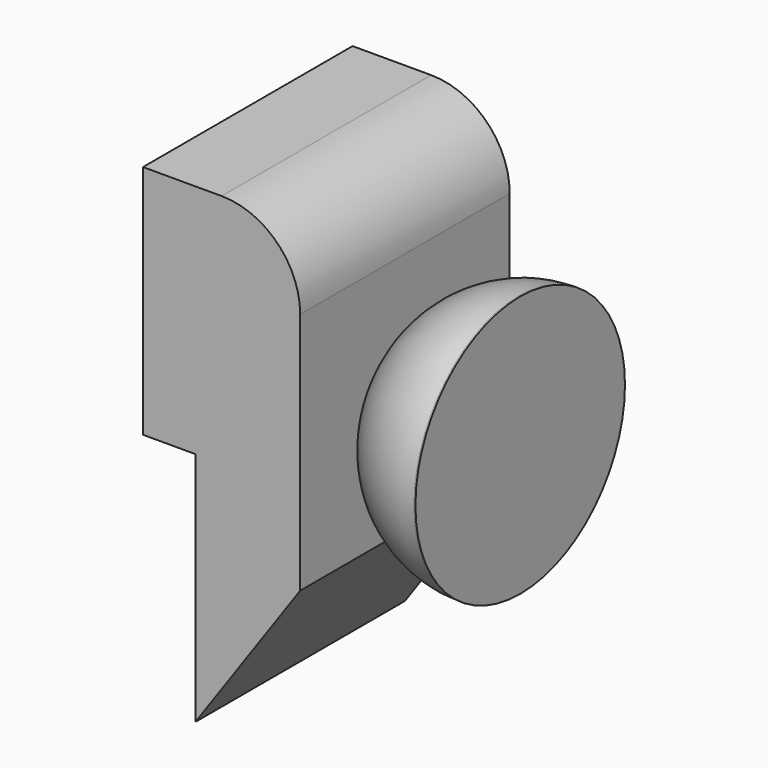
from build123d import *

# Parameters (mm, degrees)
F0_W      = 127
F0_H      = 228.6
F1_DEPTH  = 50.8
F2_R      = 38.1
F3_SIZE2  = 72.549909
F3_SIZE   = 50.79999
F4_W      = 127
F4_H      = 12.7
F5_DEPTH  = 25.4
F6_W      = 127
F6_H      = 101.6
F7_DEPTH  = 25.4
F8_R      = 25.4
F9_DEPTH  = 1.27
F10_R     = 63.5
F11_DEPTH = 54.61


# Not quite as in the source:
# - a fillet or chamfer that OpenCascade refuses, or shapes differently, is made with other operations: its cross-section is extruded or revolved along the edge and cut away or added
# - a fillet or chamfer is up to 0.001 mm smaller than in the source, because OpenCascade refuses the exact size


with BuildPart() as f1:
    # F0 (on Right) → F1 (new body)
    with BuildSketch(Plane.YZ):
        Rectangle(F0_W, F0_H)
    extrude(amount=F1_DEPTH)

    # F2
    f2_edges = [f1.edges().sort_by_distance(p)[0] for p in [
        (50.8, 0, 114.3),
    ]]
    fillet(f2_edges, radius=F2_R)

    # F3 (size 50.8 and 72.5499187425 in the source; OpenCascade refuses exactly that, so slightly less here)
    f3_edges = [f1.edges().sort_by_distance(p)[0] for p in [
        (50.8, 0, -114.3),
    ]]
    f3_side = f1.faces().sort_by_distance((25.4, 0, -114.3))[0]
    chamfer(f3_edges, length=F3_SIZE, length2=F3_SIZE2, reference=f3_side)

    # F4 (on face) → F5 (join)
    with BuildSketch(Plane(origin=(0, 0, 0), x_dir=(0, -1, 0), z_dir=(-1, 0, 0))):
        with Locations((0, 107.95)):
            Rectangle(F4_W, F4_H)
    extrude(amount=F5_DEPTH)

    # F6 (on face) → F7 (join)
    with BuildSketch(Plane(origin=(0, 0, 0), x_dir=(0, -1, 0), z_dir=(-1, 0, 0))):
        with Locations((0, 50.8)):
            Rectangle(F6_W, F6_H)
    extrude(amount=F7_DEPTH)

    # F8 (on face) → F9 (join)
    with BuildSketch(Plane.YZ.offset(50.8)):
        with Locations((0, 12.7)):
            Circle(F8_R)
    extrude(amount=F9_DEPTH)

    # F10 (on face) → F11 (join)
    with BuildSketch(Plane.YZ.offset(52.07)):
        with Locations((0, 12.7)):
            Circle(F10_R)
    extrude(amount=F11_DEPTH)

    # F12: fillet of radius 57.15 on 1 edges, made by hand

    # F12_s1 → F12_t2 (revolve, cut)
    with BuildSketch(Plane.XY.offset(12.7)):
        with BuildLine():
            ThreePointArc((105.9515367264, 63.5), (72.9559688422, 53.0127796), (52.07, 25.4))
            Line((52.07, 25.4), (52.07, 63.5))
            Line((52.07, 63.5), (105.9515367264, 63.5))
        make_face()
    revolve(axis=Axis((52.07, 0, 12.7), (1, 0, 0)), mode=Mode.SUBTRACT)


solid = f1.part
